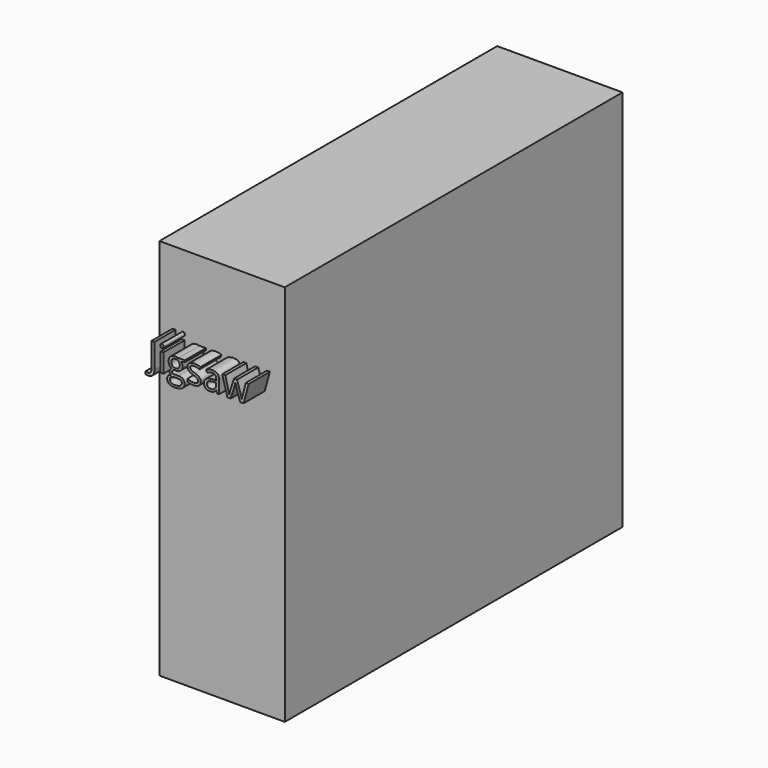
from build123d import *

# Parameters (mm, degrees)
F0_W         = 120.65
F0_H         = 368.3
F1_DEPTH     = 406.4
F2_TEXT_SIZE = 33.7436429683
F3_DEPTH     = 25.4


# Not quite as in the source:
# - Text() gives the source's letters only with a copy of the font that has no kerning and outlines rounded to 1/6400 em; it was checked with that copy


with BuildPart() as f1:
    # F0 (on Front) → F1 (new body)
    with BuildSketch(Plane.XZ):
        Rectangle(F0_W, F0_H)
    extrude(amount=F1_DEPTH)

    # F2 (on face) → F3 (join)
    with BuildSketch(Plane.XZ.offset(406.4)):
        with Locations((-50.8, 89.872049327)):
            Text('Jigsaw', F2_TEXT_SIZE, font='Open Sans', text_align=(TextAlign.LEFT, TextAlign.BOTTOM))
    extrude(amount=F3_DEPTH)


solid = f1.part
